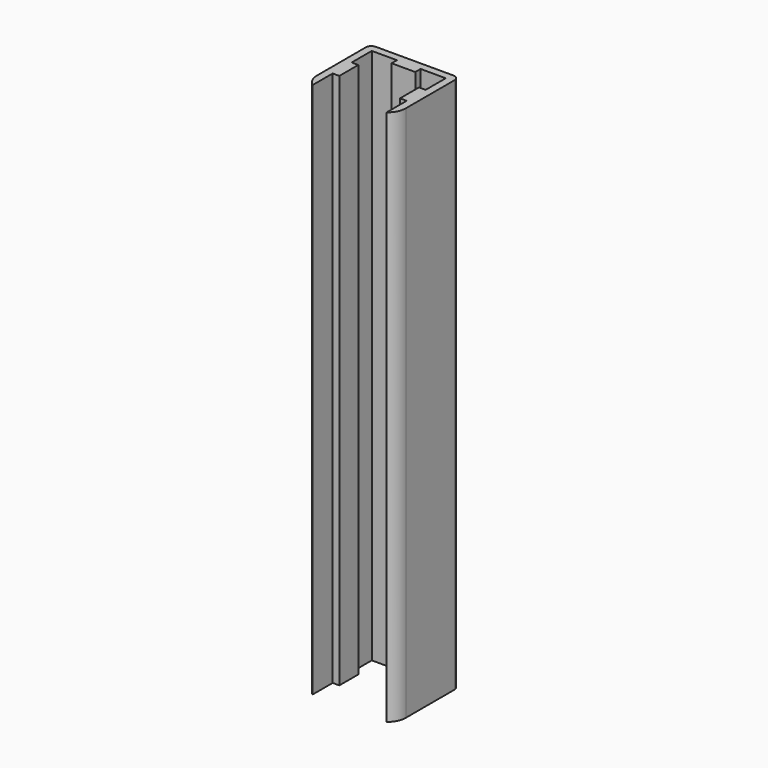
from build123d import *

# Parameters (mm, degrees)
F1_DEPTH    = 145
F2_T1_DEPTH = 165
F3_R        = 1.5


# Not quite as in the source:
# - a fillet or chamfer that OpenCascade refuses, or shapes differently, is made with other operations: its cross-section is extruded or revolved along the edge and cut away or added


with BuildPart() as f1:
    # F0 (on Top) → F1 (new body)
    with BuildSketch(Plane.XY):
        Polygon((8.4283615947, -32.4416384101), (10.4283615947, -32.4416384101), (10.4283615947, -25.6416384101), (12.2283615947, -25.6416384101), (12.2283615947, -19.2416384101), (10.4283615947, -19.2416384101), (10.4283615947, -12.4416384101), (17.2283615947, -12.4416384101), (17.2283615947, -14.2416384101), (23.6283615947, -14.2416384101), (23.6283615947, -12.4416384101), (30.4283615947, -12.4416384101), (30.4283615947, -19.2416384101), (28.6283615947, -19.2416384101), (28.6283615947, -25.6416384101), (30.4283615947, -25.6416384101), (30.4283615947, -32.4416384101), (32.4283615947, -32.4416384101), (32.4283615947, -10.4416384101), (8.4283615947, -10.4416384101), align=None)
    extrude(amount=F1_DEPTH)

    # F2: fillet of radius 5 on 2 edges, made by hand

    # F2_s2 → F2_t1 (cut)
    with BuildSketch(Plane.XY.offset(-10)):
        with BuildLine():
            ThreePointArc((8.4283615947, -28.4416384101), (8.9562256397, -30.6777063876), (10.4283615947, -32.4416384101))
            Line((10.4283615947, -32.4416384101), (8.4283615947, -32.4416384101))
            Line((8.4283615947, -32.4416384101), (8.4283615947, -28.4416384101))
        make_face()
        with BuildLine():
            ThreePointArc((30.4283615947, -32.4416384101), (31.9004975497, -30.6777063876), (32.4283615947, -28.4416384101))
            Line((32.4283615947, -28.4416384101), (32.4283615947, -32.4416384101))
            Line((32.4283615947, -32.4416384101), (30.4283615947, -32.4416384101))
        make_face()
    extrude(amount=F2_T1_DEPTH, mode=Mode.SUBTRACT)

    # F3
    f3_edges = [f1.edges().sort_by_distance(p)[0] for p in [
        (8.428362, -10.441638, 72.5),
        (32.428362, -10.441638, 72.5),
    ]]
    fillet(f3_edges, radius=F3_R)


solid = f1.part
